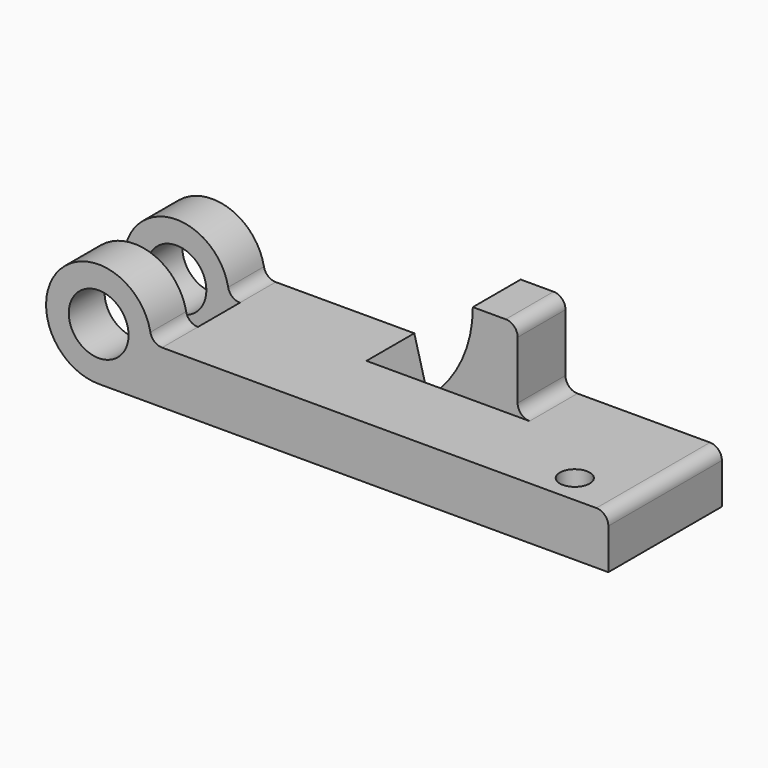
from build123d import *

# Parameters (mm, degrees)
F0_R     = 12.7
F1_DEPTH = 60.325
F2_R     = 5.08
F3_W     = 52.5957527157
F3_H     = 22.3266
F4_DEPTH = 25.908
F5_DEPTH = 25.4
F6_DEPTH = 25.4
F7_R     = 5.08
F8_R     = 6.35
F9_DEPTH = 25.4


with BuildPart() as f1:
    # F0 (on Front) → F1 (new body)
    with BuildSketch(Plane.XZ):
        with BuildLine():
            ThreePointArc((-45.2591143548, -22.352), (-29.4538635818, -15.8052507731), (-22.9071143548, 0))
            ThreePointArc((-22.9071143548, 0), (-61.0643651279, 15.8052507731), (-45.2591143548, -22.352))
        make_face()
        with Locations((-45.2591143548, 0)):
            Circle(F0_R, mode=Mode.SUBTRACT)
        Polygon((104.8294856452, 0), (71.9872856452, 0), (71.9872856452, -22.352), (171.3012856452, -22.352), (171.3012856452, 0), align=None)
        with BuildLine():
            Line((40.5928856452, 0), (-22.9071143548, 0))
            ThreePointArc((-22.9071143548, 0), (-29.4538635818, -15.8052507731), (-45.2591143548, -22.352))
            Line((-45.2591143548, -22.352), (46.5366914868, -22.352))
            Line((46.5366914868, -22.352), (40.5928856452, 0))
        make_face()
        Polygon((71.9872856452, 0), (40.5928856452, 0), (46.5366914868, -22.352), (71.9872856452, -22.352), align=None)
    extrude(amount=F1_DEPTH)

    # F2
    f2_edges = [f1.edges().sort_by_distance(p)[0] for p in [
        (-22.907114, -30.1625, 0),
        (171.301286, -30.1625, 0),
    ]]
    fillet(f2_edges, radius=F2_R)

    # F3 (on face) → F4 (cut, symmetric)
    with BuildSketch(Plane.XY):
        with Locations((-44.5994644167, -30.1625)):
            Rectangle(F3_W, F3_H)
    extrude(amount=F4_DEPTH, both=True, mode=Mode.SUBTRACT)

    # F0 (on Front) → F5 (join)
    with BuildSketch(Plane.XZ):
        with BuildLine():
            ThreePointArc((85.7794856452, 34.798), (82.2053010067, 16.0823576341), (71.9872856452, 0))
            Line((71.9872856452, 0), (104.8294856452, 0))
            Line((104.8294856452, 0), (104.8294856452, 34.798))
            Line((104.8294856452, 34.798), (85.7794856452, 34.798))
        make_face()
    extrude(amount=F5_DEPTH)

    # F0 (on Front) → F6 (cut)
    with BuildSketch(Plane.XZ):
        Polygon((71.9872856452, 0), (40.5928856452, 0), (46.5366914868, -22.352), (71.9872856452, -22.352), align=None)
    extrude(amount=F6_DEPTH, mode=Mode.SUBTRACT)

    # F7
    f7_edges = [f1.edges().sort_by_distance(p)[0] for p in [
        (104.829486, -12.7, 0),
        (104.829486, -12.7, 34.798),
    ]]
    fillet(f7_edges, radius=F7_R)

    # F8 (on face) → F9 (cut)
    with BuildSketch(Plane.XY):
        with Locations((147.1694111824, -47.9711517692)):
            Circle(F8_R)
    extrude(amount=-F9_DEPTH, mode=Mode.SUBTRACT)


solid = f1.part
